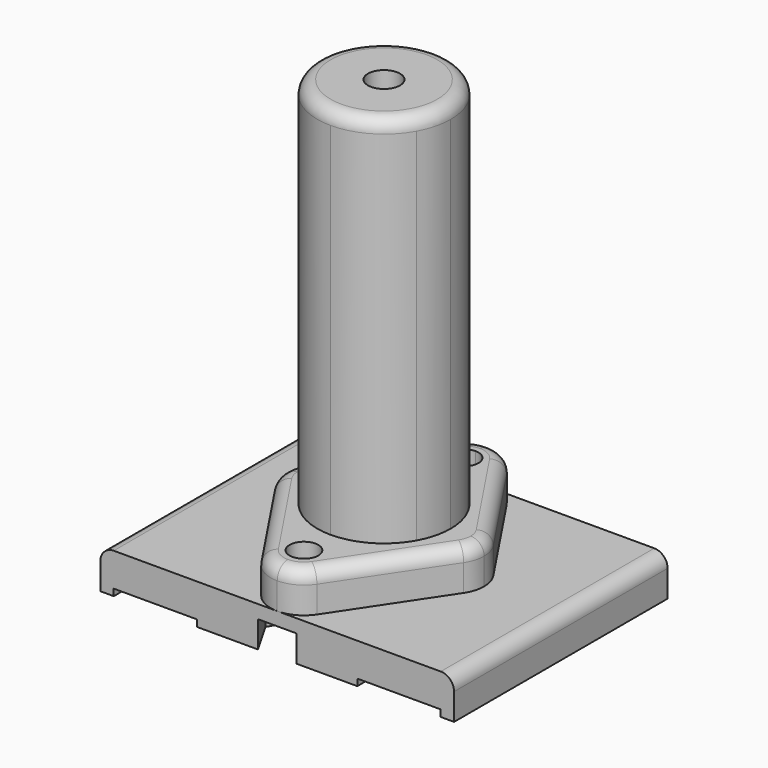
from build123d import *

# Parameters (mm, degrees)
F0_W      = 7.9375
F0_H      = 12.7
F1_DEPTH  = 3.81
F2_DEPTH  = 0.635
F3_R      = 3.9878
F3_R_2    = 2.54
F4_DEPTH  = 3.81
F6_DEPTH  = 3.81
F8_DEPTH  = 2.54
F9_W      = 12.7
F9_H      = 3.81
F10_DEPTH = 9.525
F12_DEPTH = 3.81
F14_DEPTH = 3.81
F16_DEPTH = 35.56
F17_R     = 1.27
F17_2_R   = 1.27
F18_R     = 5.2496341023
F19_DEPTH = 36.83
F20_R     = 1.524
F21_DEPTH = 25.4


# Not quite as in the source:
# - a fillet or chamfer that OpenCascade refuses, or shapes differently, is made with other operations: its cross-section is extruded or revolved along the edge and cut away or added


with BuildPart() as f1:
    # F0 (on Top) → F1 (new body)
    with BuildSketch(Plane.XY):
        Polygon((-15.5575, -12.7), (-15.5575, 0), (-15.5575, 12.7), (-16.8275, 12.7), (-16.8275, -12.7), align=None)
        with Locations((-11.58875, 6.35)):
            Rectangle(F0_W, F0_H)
        with Locations((-11.58875, -6.35)):
            Rectangle(F0_W, F0_H)
        with BuildLine():
            ThreePointArc((0, -2.54), (-1.7960512242, -1.7960512242), (-2.54, 0))
            Line((-2.54, 0), (-7.62, 0))
            Line((-7.62, 0), (-7.62, -12.7))
            Line((-7.62, -12.7), (0, -12.7))
            Line((0, -12.7), (0, -2.54))
        make_face()
        with BuildLine():
            ThreePointArc((-2.54, 0), (0, 2.54), (2.54, 0))
            Line((2.54, 0), (7.62, 0))
            Line((7.62, 0), (7.62, 12.7))
            Line((7.62, 12.7), (-7.62, 12.7))
            Line((-7.62, 12.7), (-7.62, 0))
            Line((-7.62, 0), (-2.54, 0))
        make_face()
        with BuildLine():
            Line((7.62, 0), (2.54, 0))
            ThreePointArc((2.54, 0), (1.7960512242, -1.7960512242), (0, -2.54))
            Line((0, -2.54), (0, -12.7))
            Line((0, -12.7), (7.62, -12.7))
            Line((7.62, -12.7), (7.62, 0))
        make_face()
        with Locations((11.58875, -6.35)):
            Rectangle(F0_W, F0_H)
        with Locations((11.58875, 6.35)):
            Rectangle(F0_W, F0_H)
        Polygon((15.5575, 12.7), (15.5575, 0), (15.5575, -12.7), (16.8275, -12.7), (16.8275, 12.7), align=None)
    extrude(amount=F1_DEPTH)

    # F0 (on Top) → F2 (cut)
    with BuildSketch(Plane.XY):
        with Locations((-11.58875, -6.35)):
            Rectangle(F0_W, F0_H)
        with Locations((-11.58875, 6.35)):
            Rectangle(F0_W, F0_H)
        with Locations((11.58875, 6.35)):
            Rectangle(F0_W, F0_H)
        with Locations((11.58875, -6.35)):
            Rectangle(F0_W, F0_H)
    extrude(amount=F2_DEPTH, mode=Mode.SUBTRACT)

    # F3 (on face) → F4 (cut, through all)
    with BuildSketch(Plane.XY.offset(3.81)):
        Circle(F3_R)
        Circle(F3_R_2, mode=Mode.SUBTRACT)
    extrude(amount=-F4_DEPTH, mode=Mode.SUBTRACT)

    # F5 (on face) → F6 (cut, through all)
    with BuildSketch(Plane.XY.offset(3.81)):
        with BuildLine():
            ThreePointArc((0, 10.8966), (-1.3716, 9.525), (0, 8.1534))
            Line((0, 8.1534), (0, 9.525))
            Line((0, 9.525), (0, 10.8966))
        make_face()
        with BuildLine():
            Line((0, 9.525), (0, 8.1534))
            ThreePointArc((0, 8.1534), (0.9698676611, 8.5551323389), (1.3716, 9.525))
            ThreePointArc((1.3716, 9.525), (0.9698676611, 10.4948676611), (0, 10.8966))
            Line((0, 10.8966), (0, 9.525))
        make_face()
        with BuildLine():
            ThreePointArc((1.3716, -9.525), (0.9698676611, -8.5551323389), (0, -8.1534))
            Line((0, -8.1534), (0, -9.525))
            Line((0, -9.525), (0, -10.8966))
            ThreePointArc((0, -10.8966), (0.9698676611, -10.4948676611), (1.3716, -9.525))
        make_face()
        with BuildLine():
            Line((0, -9.525), (0, -8.1534))
            ThreePointArc((0, -8.1534), (-1.3716, -9.525), (0, -10.8966))
            Line((0, -10.8966), (0, -9.525))
        make_face()
    extrude(amount=-F6_DEPTH, mode=Mode.SUBTRACT)

    # F7 (on face) → F8 (cut)
    with BuildSketch(Plane.XY):
        Polygon((1.8330871047, -6.35), (0, -6.35), (0, -9.525), (0, -12.7), (1.8330871047, -12.7), (3.6661742094, -9.525), align=None)
        Polygon((0, -12.7), (0, -9.525), (-3.6661742094, -9.525), (-1.8330871047, -12.7), align=None)
        Polygon((0, -9.525), (0, -6.35), (-1.8330871047, -6.35), (-3.6661742094, -9.525), align=None)
        Polygon((0, 9.525), (0, 6.35), (1.8330871047, 6.35), (3.6661742094, 9.525), (1.8330871047, 12.7), (-1.8330871047, 12.7), (-3.6661742094, 9.525), align=None)
        Polygon((-1.8330871047, 6.35), (0, 6.35), (0, 9.525), (-3.6661742094, 9.525), align=None)
    extrude(amount=F8_DEPTH, mode=Mode.SUBTRACT)

    # F17
    f17_edges = [f1.edges().sort_by_distance(p)[0] for p in [
        (16.8275, 0, 3.81),
        (-16.8275, 0, 3.81),
    ]]
    fillet(f17_edges, radius=F17_R)


with BuildPart() as f10:
    # F9 (on Right) → F10 (new body, symmetric)
    with BuildSketch(Plane.YZ):
        with Locations((6.35, 5.715)):
            Rectangle(F9_W, F9_H)
        with Locations((-6.35, 5.715)):
            Rectangle(F9_W, F9_H)
    extrude(amount=F10_DEPTH, both=True)

    # F11 (on face) → F12 (cut)
    with BuildSketch(Plane.XY.offset(7.62)):
        with BuildLine():
            ThreePointArc((1.3716, 9.525), (0.9698676611, 10.4948676611), (0, 10.8966))
            ThreePointArc((0, 10.8966), (-0.9698676611, 8.5551323389), (1.3716, 9.525))
        make_face()
        with BuildLine():
            ThreePointArc((1.3716, -9.525), (-0.9698676611, -8.5551323389), (0, -10.8966))
            ThreePointArc((0, -10.8966), (0.9698676611, -10.4948676611), (1.3716, -9.525))
        make_face()
    extrude(amount=-F12_DEPTH, mode=Mode.SUBTRACT)

    # F13 (on face) → F14 (cut)
    with BuildSketch(Plane.XY.offset(7.62)):
        with BuildLine():
            Line((-8.9917596845, 1.761173123), (-2.6417596845, 11.286173123))
            ThreePointArc((-2.6417596845, 11.286173123), (-1.4981489136, 12.3243168511), (0, 12.7))
            Line((0, 12.7), (-9.525, 12.7))
            Line((-9.525, 12.7), (-9.525, 0))
            ThreePointArc((-9.525, 0), (-9.3887671841, 0.9200646721), (-8.9917596845, 1.761173123))
        make_face()
        with BuildLine():
            ThreePointArc((0, 12.7), (1.4981489136, 12.3243168511), (2.6417596845, 11.286173123))
            Line((2.6417596845, 11.286173123), (8.9917596845, 1.761173123))
            ThreePointArc((8.9917596845, 1.761173123), (9.3887671841, 0.9200646721), (9.525, 0))
            Line((9.525, 0), (9.525, 12.7))
            Line((9.525, 12.7), (0, 12.7))
        make_face()
        with BuildLine():
            ThreePointArc((-8.9917596845, -1.761173123), (-9.3887671841, -0.9200646721), (-9.525, 0))
            Line((-9.525, 0), (-9.525, -12.7))
            Line((-9.525, -12.7), (-2.72e-08, -12.7))
            ThreePointArc((-2.72e-08, -12.7), (-1.4981489256, -12.3243168447), (-2.6417596845, -11.286173123))
            Line((-2.6417596845, -11.286173123), (-8.9917596845, -1.761173123))
        make_face()
        with BuildLine():
            Line((9.525, -12.7), (9.525, 0))
            ThreePointArc((9.525, 0), (9.3887671841, -0.9200646721), (8.9917596845, -1.761173123))
            Line((8.9917596845, -1.761173123), (2.6417596845, -11.286173123))
            ThreePointArc((2.6417596845, -11.286173123), (1.4981489016, -12.3243168575), (-2.72e-08, -12.7))
            Line((-2.72e-08, -12.7), (9.525, -12.7))
        make_face()
    extrude(amount=-F14_DEPTH, mode=Mode.SUBTRACT)

    # F15 (on face) → F16 (join)
    with BuildSketch(Plane.XY.offset(7.62)):
        with BuildLine():
            ThreePointArc((-3.175, 0), (-3.8399421072, 1.9442824833), (-5.55625, 3.0741805311))
            ThreePointArc((-5.55625, 3.0741805311), (-6.35, 0), (-5.55625, -3.0741805311))
            ThreePointArc((-5.55625, -3.0741805311), (-3.8399421072, -1.9442824833), (-3.175, 0))
        make_face()
        with BuildLine():
            Line((0, 0), (0, 6.35))
            ThreePointArc((-1.01e-08, 6.35), (-3.2250157894, 5.4700798128), (-5.55625, 3.0741805311))
            ThreePointArc((-5.55625, 3.0741805311), (-3.8399421072, 1.9442824833), (-3.175, 0))
            ThreePointArc((-3.175, 0), (-3.8399421072, -1.9442824833), (-5.55625, -3.0741805311))
            ThreePointArc((-5.55625, -3.0741805311), (-3.2250157851, -5.4700798153), (0, -6.35))
            Line((0, -6.35), (0, 0))
        make_face()
        with BuildLine():
            ThreePointArc((5.55625, -3.0741805311), (3.175, 0), (5.55625, 3.0741805311))
            ThreePointArc((5.55625, 3.0741805311), (3.2250157807, 5.4700798179), (-1.01e-08, 6.35))
            Line((0, 6.35), (0, 0))
            Line((0, 0), (0, -6.35))
            ThreePointArc((0, -6.35), (3.2250157851, -5.4700798153), (5.55625, -3.0741805311))
        make_face()
        with BuildLine():
            ThreePointArc((5.55625, -3.0741805311), (6.1483610621, -1.5875), (6.35, 0))
            ThreePointArc((6.35, 0), (6.1483610621, 1.5875), (5.55625, 3.0741805311))
            ThreePointArc((5.55625, 3.0741805311), (3.175, 0), (5.55625, -3.0741805311))
        make_face()
    extrude(amount=F16_DEPTH)

    # F17#2
    f17_2_edges = [f10.edges().sort_by_distance(p)[0] for p in [
        (5.81676, -6.523673, 7.62),
    ]]
    fillet(f17_2_edges, radius=F17_2_R)

    # F18 (on face) → F19 (cut)
    with BuildSketch(Plane(origin=(0, 0, 3.81), x_dir=(1, 0, 0), z_dir=(0, 0, -1))):
        Circle(F18_R)
    extrude(amount=-F19_DEPTH, mode=Mode.SUBTRACT)

    # F20 (on face) → F21 (cut)
    with BuildSketch(Plane.XY.offset(43.18)):
        Circle(F20_R)
    extrude(amount=-F21_DEPTH, mode=Mode.SUBTRACT)

    # F22: fillet of radius 1.27 on 1 edges, made by hand

    # F22_s1 → F22_t2 (revolve, cut)
    with BuildSketch(Plane.YZ):
        with BuildLine():
            ThreePointArc((6.35, 41.91), (5.9780256121, 42.8080256121), (5.08, 43.18))
            Line((5.08, 43.18), (6.35, 43.18))
            Line((6.35, 43.18), (6.35, 41.91))
        make_face()
    revolve(axis=Axis((0, 0, 43.18), (0, 0, -1)), mode=Mode.SUBTRACT)


solid = Compound([f1.part, f10.part])
